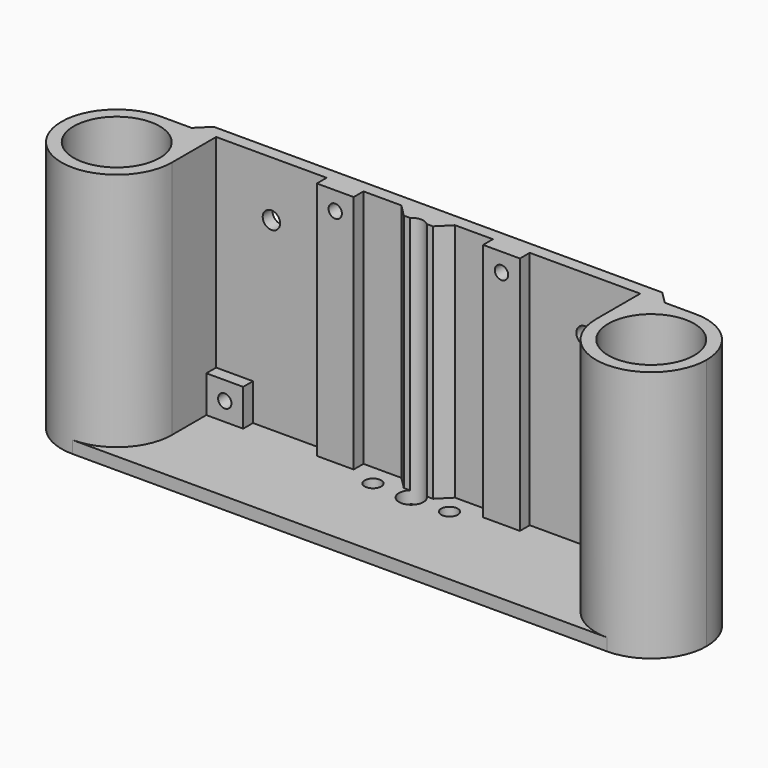
from build123d import *

# Parameters (mm, degrees)
F0_R      = 11.1125
F1_DEPTH  = 65.211198
F3_DEPTH  = 3.175
F4_R      = 14.28749
F5_R      = 2.2479
F5_R_2    = 1.7272
F6_DEPTH  = 6.35
F7_R      = 3.175
F7_R_2    = 2.15265
F8_DEPTH  = 65.211198
F9_W      = 12.9742907321
F9_H      = 62.036198
F10_DEPTH = 3.175
F11_SIZE  = 3.17499


# Not quite as in the source:
# - a fillet or chamfer is up to 0.001 mm smaller than in the source, because OpenCascade refuses the exact size
# - a feature names something its author has since deleted; it is built from what else it names


with BuildPart() as f1:
    # F0 (on Top) → F1 (new body)
    with BuildSketch(Plane.XY):
        with BuildLine():
            Line((22.225, 0), (0, 0))
            Line((0, 0), (0, -14.2875))
            ThreePointArc((0, -14.2875), (14.2875, -28.575), (28.575, -14.2875))
            Line((28.575, -14.2875), (28.575, -3.175))
            Line((28.575, -3.175), (138.2559846, -3.175))
            Line((138.2559846, -3.175), (138.2559846, -14.2875))
            ThreePointArc((138.2559846, -14.2875), (152.5434846, -28.575), (166.8309846, -14.2875))
            Line((166.8309846, -14.2875), (166.8309846, 0))
            Line((166.8309846, 0), (144.6059846, 0))
            Line((144.6059846, 0), (144.6059846, 3.175))
            Line((144.6059846, 3.175), (22.225, 3.175))
            Line((22.225, 3.175), (22.225, 0))
        make_face()
        with Locations((14.2875, -14.2875)):
            Circle(F0_R, mode=Mode.SUBTRACT)
        with Locations((152.5434846, -14.2875)):
            Circle(F0_R, mode=Mode.SUBTRACT)
    extrude(amount=F1_DEPTH)

    # F2 (on face) → F3 (join)
    with BuildSketch(Plane(origin=(0, 0, 0), x_dir=(1, 0, 0), z_dir=(0, 0, -1))):
        with BuildLine():
            Line((152.5434846, 28.575), (14.2875, 28.575))
            ThreePointArc((14.2875, 28.575), (24.3902881362, 24.3902881362), (28.575, 14.2875))
            Line((28.575, 14.2875), (28.575, 3.175))
            Line((28.575, 3.175), (138.2559846, 3.175))
            Line((138.2559846, 3.175), (138.2559846, 14.2875))
            ThreePointArc((138.2559846, 14.2875), (142.4406964638, 24.3902881362), (152.5434846, 28.575))
        make_face()
    extrude(amount=-F3_DEPTH)

    # F4 (radius 14.2875 in the source; OpenCascade refuses exactly that, so slightly less here)
    f4_edges = [f1.edges().sort_by_distance(p)[0] for p in [
        (0, 0, 32.605599),
        (166.830985, 0, 32.605599),
    ]]
    fillet(f4_edges, radius=F4_R)

    # F5 (on face) → F6 (cut, through all)
    with BuildSketch(Plane(origin=(0, 3.175, 0), x_dir=(-1, 0, 0), z_dir=(0, 1, 0))):
        with Locations((-123.9684846, 50.923698)):
            Circle(F5_R)
        with Locations((-104.9184846, 60.448698)):
            Circle(F5_R_2)
        with Locations((-61.9125, 60.448698)):
            Circle(F5_R_2)
        with Locations((-42.8625, 50.923698)):
            Circle(F5_R)
        with Locations((-133.4934846, 7.9375)):
            Circle(F5_R_2)
        with Locations((-33.3375, 7.9375)):
            Circle(F5_R_2)
    extrude(amount=-F6_DEPTH, mode=Mode.SUBTRACT)

    # F7 (on face) → F8 (cut, through all)
    with BuildSketch(Plane(origin=(0, 0, 0), x_dir=(1, 0, 0), z_dir=(0, 0, -1))):
        with Locations((83.4154923, 5.4845204)):
            Circle(F7_R)
        with Locations((73.5203484069, 5.4845204)):
            Circle(F7_R_2)
        with Locations((93.3106361931, 5.4845204)):
            Circle(F7_R_2)
    extrude(amount=-F8_DEPTH, mode=Mode.SUBTRACT)

    # F9 (on face) → F10 (cut)
    with BuildSketch(Plane.XZ.offset(3.175)):
        Polygon((57.15, 65.211198), (28.575, 65.211198), (28.575, 12.7), (38.1, 12.7), (38.1, 3.175), (57.15, 3.175), align=None)
        Polygon((138.2559846, 12.7), (138.2559846, 65.211198), (109.6809846, 65.211198), (109.6809846, 3.175), (128.7309846, 3.175), (128.7309846, 12.7), align=None)
        with Locations((73.162145366, 34.193099)):
            Rectangle(F9_W, F9_H)
        with Locations((93.668839234, 34.193099)):
            Rectangle(F9_W, F9_H)
    extrude(amount=-F10_DEPTH, mode=Mode.SUBTRACT)

    # F11 (size 3.175 in the source; OpenCascade refuses exactly that, so slightly less here)
    f11_edges = [f1.edges().sort_by_distance(p)[0] for p in [
        (22.225, 3.175, 32.605599),
        (144.605985, 3.175, 32.605599),
        (87.181694, 0, 34.193099),
        (79.649291, 0, 34.193099),
    ]]
    chamfer(f11_edges, length=F11_SIZE)


solid = f1.part
